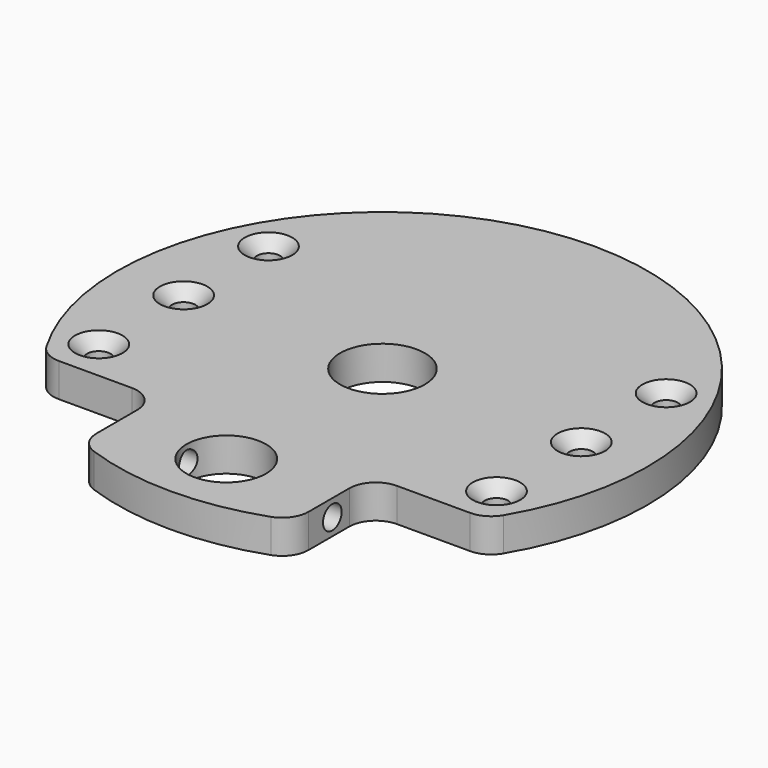
from build123d import *

# Parameters (mm, degrees)
F0_R           = 50
F1_DEPTH       = 6.35
F3_D           = 4.4
F3_CSINK_D     = 8.96
F3_CSINK_ANGLE = 90
F4_R           = 8
F5_DEPTH       = 8
F7_DEPTH       = 25
F9_R           = 5
F10_D          = 4.4
F11_R          = 7.5
F12_DEPTH      = 25


# Not quite as in the source:
# - a feature names something its author has since deleted; it is built from what else it names


with BuildPart() as f1:
    # F0 (on Top) → F1 (new body)
    with BuildSketch(Plane.XY):
        Circle(F0_R)
    extrude(amount=F1_DEPTH)

    # F3 (through all)
    with Locations(Plane.XY.offset(6.35)):
        with Locations((-37.5, 20), (-37.5, 0), (-37.5, -20), (37.5, 20), (37.5, 0), (37.5, -20)):
            CounterSinkHole(F3_D / 2, F3_CSINK_D / 2, counter_sink_angle=F3_CSINK_ANGLE)

    # F4 (on face) → F5 (cut)
    with BuildSketch(Plane.XY.offset(6.35)):
        Circle(F4_R)
    extrude(amount=-F5_DEPTH, mode=Mode.SUBTRACT)

    # F6 (on face) → F7 (cut)
    with BuildSketch(Plane.XY.offset(6.35)):
        with BuildLine():
            Line((-20, -27.8257569496), (-41.5418734554, -27.8257569496))
            ThreePointArc((-41.5418734554, -27.8257569496), (-32.0601083451, -38.3685998298), (-20, -45.8257569496))
            Line((-20, -45.8257569496), (-20, -27.8257569496))
        make_face()
        with BuildLine():
            ThreePointArc((20, -45.8257569496), (32.0601083451, -38.3685998298), (41.5418734554, -27.8257569496))
            Line((41.5418734554, -27.8257569496), (20, -27.8257569496))
            Line((20, -27.8257569496), (20, -45.8257569496))
        make_face()
    extrude(amount=-F7_DEPTH, mode=Mode.SUBTRACT)

    # F9
    f9_edges = [f1.edges().sort_by_distance(p)[0] for p in [
        (-41.541873, -27.825757, 3.175),
        (-20, -45.825757, 3.175),
        (-20, -27.825757, 3.175),
        (20, -27.825757, 3.175),
        (20, -45.825757, 3.175),
        (41.541873, -27.825757, 3.175),
    ]]
    fillet(f9_edges, radius=F9_R)

    # F10 (through all)
    with Locations(Plane.YZ.offset(20)):
        with Locations((-36.8257569496, 3.175)):
            Hole(F10_D / 2)

    # F11 (on face) → F12 (cut)
    with BuildSketch(Plane.XY.offset(6.35)):
        with Locations((0, -36.8257569496)):
            Circle(F11_R)
    extrude(amount=-F12_DEPTH, mode=Mode.SUBTRACT)


solid = f1.part
